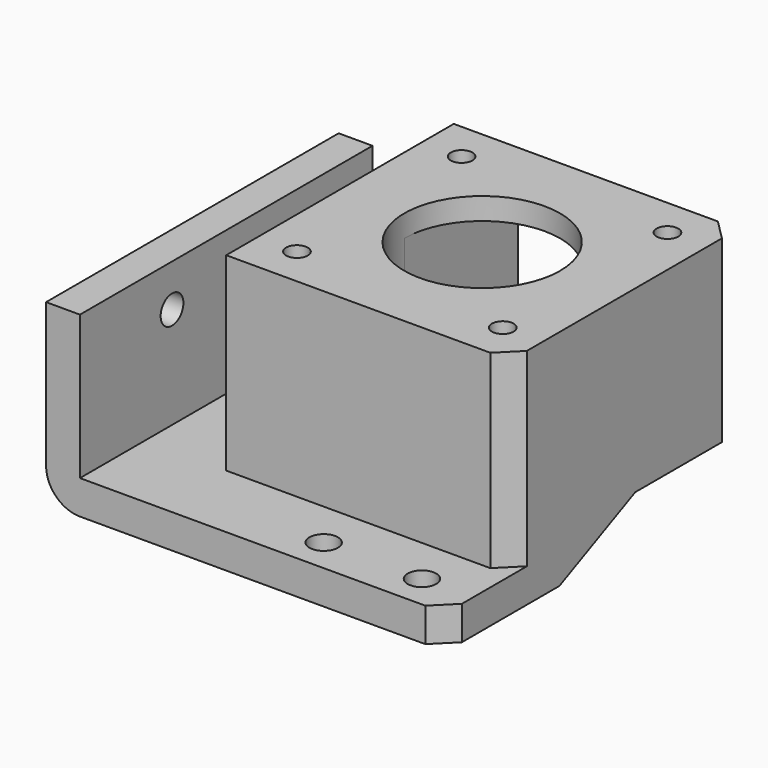
from build123d import *

# Parameters (mm, degrees)
F0_W      = 59
F0_H      = 54
F1_DEPTH  = 5
F2_W      = 5
F2_H      = 54
F3_DEPTH  = 21.25
F4_W      = 42
F4_H      = 42
F5_DEPTH  = 28
F6_R      = 1.6
F6_R_2    = 11.5
F7_DEPTH  = 33.001
F8_R      = 2.1
F9_DEPTH  = 5.001
F10_W     = 23
F10_H     = 15
F11_DEPTH = 21.001
F13_DEPTH = 33
F14_SIZE  = 3
F16_DEPTH = 10.6937211186
F17_R     = 5
F18_R     = 1.6
F19_DEPTH = 8.25
F20_R     = 1.6
F21_DEPTH = 2.5
F22_R     = 2.1
F23_DEPTH = 5


with BuildPart() as f1:
    # F0 (on Top) → F1 (new body)
    with BuildSketch(Plane.XY):
        with Locations((29.5, 27)):
            Rectangle(F0_W, F0_H)
    extrude(amount=F1_DEPTH)

    # F2 (on face) → F3 (join)
    with BuildSketch(Plane.XY.offset(5)):
        with Locations((2.5, 27)):
            Rectangle(F2_W, F2_H)
    extrude(amount=F3_DEPTH)

    # F4 (on face) → F5 (join)
    with BuildSketch(Plane.XY.offset(5)):
        with Locations((38, 33)):
            Rectangle(F4_W, F4_H)
    extrude(amount=F5_DEPTH)

    # F6 (on face) → F7 (cut, through all)
    with BuildSketch(Plane.XY.offset(33)):
        with Locations((22.8, 48.2)):
            Circle(F6_R)
        with Locations((38, 33)):
            Circle(F6_R_2)
        with Locations((53.2, 48.2)):
            Circle(F6_R)
        with Locations((22.8, 17.8)):
            Circle(F6_R)
        with Locations((53.2, 17.8)):
            Circle(F6_R)
    extrude(amount=-F7_DEPTH, mode=Mode.SUBTRACT)

    # F8 (on face) → F9 (cut, through all)
    with BuildSketch(Plane.XY.offset(5)):
        with Locations((37, 5)):
            Circle(F8_R)
        with Locations((51.5, 5)):
            Circle(F8_R)
    extrude(amount=-F9_DEPTH, mode=Mode.SUBTRACT)

    # F10 (on face) → F11 (cut, through all)
    with BuildSketch(Plane(origin=(0, 54, 0), x_dir=(-1, 0, 0), z_dir=(0, 1, 0))):
        with Locations((-38, 22.25)):
            Rectangle(F10_W, F10_H)
    extrude(amount=-F11_DEPTH, mode=Mode.SUBTRACT)

    # F12 (on face) → F13 (cut)
    with BuildSketch(Plane.YZ.offset(59)):
        Polygon((54, 0), (54, 6.5), (35, 6.5), (21, 0), align=None)
    extrude(amount=-F13_DEPTH, mode=Mode.SUBTRACT)

    # F14
    f14_edges = [f1.edges().sort_by_distance(p)[0] for p in [
        (59, 0, 2.5),
        (59, 12, 19),
        (59, 54, 19.75),
    ]]
    chamfer(f14_edges, length=F14_SIZE)

    # F15 (on face) → F16 (cut, through all)
    with BuildSketch(Plane(origin=(0, 54, 0), x_dir=(-1, 0, 0), z_dir=(0, 1, 0))):
        with BuildLine():
            Line((-32.9, 9.385948213), (-32.9031732506, 9.385948213))
            ThreePointArc((-32.9031732506, 9.385948213), (-37.0015866253, 13.6), (-41.1, 9.385948213))
            Line((-41.1, 9.385948213), (-41.1, 6.5))
            Line((-41.1, 6.5), (-32.9, 6.5))
            Line((-32.9, 6.5), (-32.9, 9.385948213))
        make_face()
    extrude(amount=-F16_DEPTH, mode=Mode.SUBTRACT)

    # F17
    f17_edges = [f1.edges().sort_by_distance(p)[0] for p in [
        (0, 27, 0),
    ]]
    fillet(f17_edges, radius=F17_R)

    # F18 (on face) → F19 (cut, through all)
    with BuildSketch(Plane(origin=(0, 0, 6.5), x_dir=(1, 0, 0), z_dir=(0, 0, -1))):
        with Locations((29.8, -48.2)):
            Circle(F18_R)
    extrude(amount=-F19_DEPTH, mode=Mode.SUBTRACT)

    # F20 (on face) → F21 (cut)
    with BuildSketch(Plane.XY.offset(14.75)):
        Polygon((31.4165807537, 45.4), (33.0331615075, 48.2), (31.4165807537, 51), (28.1834192463, 51), (26.5668384925, 48.2), (28.1834192463, 45.4), align=None)
        with Locations((29.8, 48.2)):
            Circle(F20_R, mode=Mode.SUBTRACT)
    extrude(amount=-F21_DEPTH, mode=Mode.SUBTRACT)

    # F22 (on face) → F23 (cut, through all)
    with BuildSketch(Plane(origin=(0, 0, 0), x_dir=(0, -1, 0), z_dir=(-1, 0, 0))):
        with Locations((-49, 20)):
            Circle(F22_R)
        with Locations((-17, 20)):
            Circle(F22_R)
    extrude(amount=-F23_DEPTH, mode=Mode.SUBTRACT)


solid = f1.part
